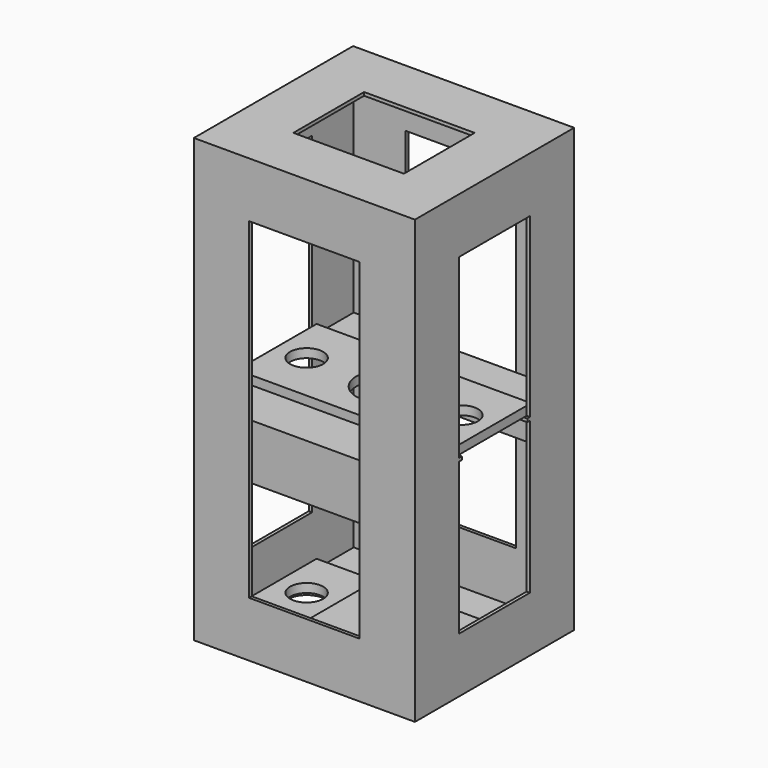
from build123d import *

# Parameters (mm, degrees)
F0_W      = 194
F0_H      = 90
F0_R      = 15
F0_R_2    = 25
F1_DEPTH  = 8
F2_W      = 80
F2_H      = 70
F3_DEPTH  = 3
F4_R      = 14
F5_DEPTH  = 25
F6_W      = 200
F6_H      = 400
F7_DEPTH  = 90
F8_W      = 100
F8_H      = 300
F9_DEPTH  = 266
F10_T     = -3
F11_W     = 80
F11_H     = 300
F12_DEPTH = 162
F13_W     = 100
F13_H     = 80
F14_DEPTH = 517
F15_R     = 17.5
F16_DEPTH = 25
F18_DEPTH = 100
F19_W     = 194
F19_H     = 90
F20_DEPTH = 8
F21_R     = 25
F21_R_2   = 15
F22_DEPTH = 25


with BuildPart() as f1:
    # F0 (on Top) → F1 (new body)
    with BuildSketch(Plane.XY):
        Rectangle(F0_W, F0_H)
        with Locations((-70, 0)):
            Circle(F0_R, mode=Mode.SUBTRACT)
        Circle(F0_R_2, mode=Mode.SUBTRACT)
        with Locations((70, 0)):
            Circle(F0_R, mode=Mode.SUBTRACT)
    extrude(amount=F1_DEPTH)


with BuildPart() as f3:
    # F2 (on face) → F3 (new body)
    with BuildSketch(Plane.XY.offset(8)):
        Rectangle(F2_W, F2_H)
    extrude(amount=F3_DEPTH)

    # F4 (on face) → F5 (cut)
    with BuildSketch(Plane.XY.offset(11)):
        Circle(F4_R)
    extrude(amount=-F5_DEPTH, mode=Mode.SUBTRACT)


with BuildPart() as f7:
    # F6 (on Front) → F7 (new body, symmetric)
    with BuildSketch(Plane.XZ):
        with Locations((0, 197)):
            Rectangle(F6_W, F6_H)
    extrude(amount=F7_DEPTH, both=True)

    # F8 (on face) → F9 (cut)
    with BuildSketch(Plane.XZ.offset(90)):
        with Locations((0, 197)):
            Rectangle(F8_W, F8_H)
    extrude(amount=-F9_DEPTH, mode=Mode.SUBTRACT)

    # F10
    f10_openings = [f7.faces().sort_by_distance(p)[0] for p in [
        (50, 0, 197),
        (0, 0, 347),
        (-50, 0, 197),
        (0, 0, 47),
    ]]
    offset(amount=F10_T, openings=f10_openings)

    # F11 (on Right) → F12 (cut, symmetric)
    with BuildSketch(Plane.YZ):
        with Locations((0, 197)):
            Rectangle(F11_W, F11_H)
    extrude(amount=F12_DEPTH, both=True, mode=Mode.SUBTRACT)

    # F13 (on face) → F14 (cut)
    with BuildSketch(Plane.XY.offset(397)):
        Rectangle(F13_W, F13_H)
    extrude(amount=-F14_DEPTH, mode=Mode.SUBTRACT)

    # F15 (on face) → F16 (cut)
    with BuildSketch(Plane(origin=(0, 0, -3), x_dir=(1, 0, 0), z_dir=(0, 0, -1))):
        with Locations((70, 0)):
            Circle(F15_R)
        with Locations((-70, 0)):
            Circle(F15_R)
    extrude(amount=-F16_DEPTH, mode=Mode.SUBTRACT)

    # F17 (on Right) → F18 (join, symmetric)
    with BuildSketch(Plane.YZ):
        Polygon((84, 184), (84, 137), (87, 137), (87, 187), (37, 187), (37, 184), align=None)
        Polygon((-87, 137), (-84, 137), (-84, 184), (-37, 184), (-37, 187), (-87, 187), align=None)
    extrude(amount=F18_DEPTH, both=True)


with BuildPart() as f20:
    # F19 (on face) → F20 (new body)
    with BuildSketch(Plane.XY.offset(187)):
        Rectangle(F19_W, F19_H)
    extrude(amount=F20_DEPTH)

    # F21 (on face) → F22 (cut)
    with BuildSketch(Plane.XY.offset(195)):
        Circle(F21_R)
        with Locations((70, 0)):
            Circle(F21_R_2)
        with Locations((-70, 0)):
            Circle(F21_R_2)
    extrude(amount=-F22_DEPTH, mode=Mode.SUBTRACT)


solid = Compound([f1.part, f3.part, f7.part, f20.part])
